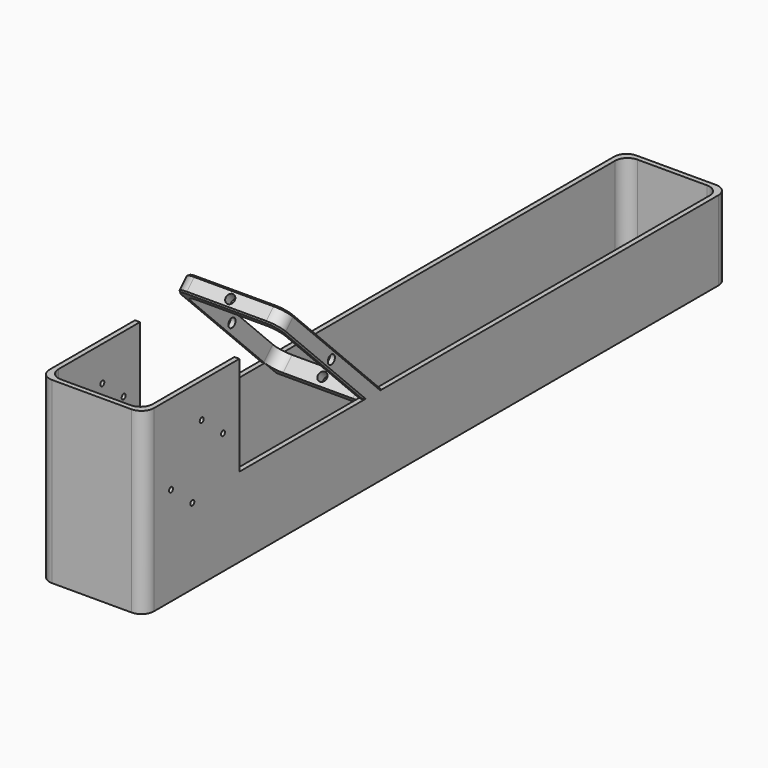
from build123d import *

# Parameters (mm, degrees)
F1_DEPTH      = 16
F3_D          = 18
F5_D          = 18
F6_ANGLE      = 45
F8_START      = -100
F8_DEPTH      = 160
F9_DEPTH      = 100
F9_DEPTH_BACK = 100
F10_T1_DEPTH  = 32
F10_T3_DEPTH  = 32
F10_T5_DEPTH  = 360
F10_T7_DEPTH  = 160
F10_T9_DEPTH  = 157
F10_T11_DEPTH = 157
F10_T13_DEPTH = 485
F10_T15_DEPTH = 285
F11_SIZE      = 3
F13_D         = 10


# Not quite as in the source:
# - a fillet or chamfer that OpenCascade refuses, or shapes differently, is made with other operations: its cross-section is extruded or revolved along the edge and cut away or added


with BuildPart() as f1:
    # F0 (on Front) → F1 (new body, symmetric)
    with BuildSketch(Plane.XZ):
        Polygon((-95, 16), (-105, 16), (-105, -16), (-105, -174), (105, -174), (105, -16), (105, 16), (95, 16), (95, -16), (95, -154), (-95, -154), (-95, -16), align=None)
        Polygon((-105, 174), (-105, 16), (-95, 16), (-95, 154), (95, 154), (95, 16), (105, 16), (105, 174), align=None)
    extrude(amount=F1_DEPTH, both=True)

    # F3 (through all)
    with Locations(Plane.YZ.offset(105)):
        with Locations((0, 0)):
            Hole(F3_D / 2)

    # F5 (through all)
    with Locations(Plane.XY.offset(174)):
        with Locations((0, 0)):
            Hole(F5_D / 2)


with BuildPart() as f1_1:
    # F6: moved
    add(f1.part.rotate(Axis((0, 0, 16), (1, 0, 0)), F6_ANGLE))

    # F7 (on Top) → F8 (join)
    with BuildSketch(Plane.XY.offset(F8_START)):
        Polygon((0, 1010), (-105, 1010), (-105, -220), (-95, -220), (-95, 1000), (0, 1000), (95, 1000), (95, -220), (105, -220), (105, 1010), align=None)
        Polygon((-95, -220), (-105, -220), (-105, -460), (0, -460), (105, -460), (105, -220), (95, -220), (95, -450), (0, -450), (-95, -450), align=None)
    extrude(amount=-F8_DEPTH)

    # F7 (on Top) → F9 (join, two sides)
    with BuildSketch(Plane.XY) as f9_sk:
        Polygon((-95, -220), (-105, -220), (-105, -460), (0, -460), (105, -460), (105, -220), (95, -220), (95, -450), (0, -450), (-95, -450), align=None)
    extrude(amount=F9_DEPTH)
    extrude(f9_sk.sketch, amount=-F9_DEPTH_BACK)

    # F10: fillet of radius 25 on 14 edges, made by hand

    # F10_s2 → F10_t1 (join)
    with BuildSketch(Plane(origin=(0, -3.313708499, -3.313708499), x_dir=(1, 0, 0), z_dir=(0, 0.7071067812, 0.7071067812))):
        with BuildLine():
            ThreePointArc((-95, 133.686291501), (-87.6776695297, 151.3639610307), (-70, 158.686291501))
            Line((-70, 158.686291501), (-95, 158.686291501))
            Line((-95, 158.686291501), (-95, 133.686291501))
        make_face()
    extrude(amount=F10_T1_DEPTH)

    # F10_s4 → F10_t3 (join)
    with BuildSketch(Plane(origin=(0, 19.313708499, 19.313708499), x_dir=(1, 0, 0), z_dir=(0, -0.7071067812, -0.7071067812))):
        with BuildLine():
            ThreePointArc((70, -158.686291501), (87.6776695297, -151.3639610307), (95, -133.686291501))
            Line((95, -133.686291501), (95, -158.686291501))
            Line((95, -158.686291501), (70, -158.686291501))
        make_face()
        with BuildLine():
            ThreePointArc((95, 124.313708499), (87.6776695297, 141.9913780286), (70, 149.313708499))
            Line((70, 149.313708499), (95, 149.313708499))
            Line((95, 149.313708499), (95, 124.313708499))
        make_face()
        with BuildLine():
            ThreePointArc((-95, 124.313708499), (-87.6776695297, 141.9913780286), (-70, 149.313708499))
            Line((-70, 149.313708499), (-95, 149.313708499))
            Line((-95, 149.313708499), (-95, 124.313708499))
        make_face()
    extrude(amount=F10_T3_DEPTH)

    # F10_s6 → F10_t5 (join)
    with BuildSketch(Plane.XY.offset(-260)):
        with BuildLine():
            ThreePointArc((-95, -425), (-87.6776695297, -442.6776695297), (-70, -450))
            Line((-70, -450), (-95, -450))
            Line((-95, -450), (-95, -425))
        make_face()
        with BuildLine():
            ThreePointArc((95, -425), (87.6776695297, -442.6776695297), (70, -450))
            Line((70, -450), (95, -450))
            Line((95, -450), (95, -425))
        make_face()
    extrude(amount=F10_T5_DEPTH)

    # F10_s8 → F10_t7 (join)
    with BuildSketch(Plane.XY.offset(-260)):
        with BuildLine():
            ThreePointArc((95, 975), (87.6776695297, 992.6776695297), (70, 1000))
            Line((70, 1000), (95, 1000))
            Line((95, 1000), (95, 975))
        make_face()
        with BuildLine():
            ThreePointArc((-95, 975), (-87.6776695297, 992.6776695297), (-70, 1000))
            Line((-70, 1000), (-95, 1000))
            Line((-95, 1000), (-95, 975))
        make_face()
    extrude(amount=F10_T7_DEPTH)

    # F10_s10 → F10_t9 (cut)
    with BuildSketch(Plane(origin=(0, 63.5078823231, 63.5078823231), x_dir=(1, 0, 0), z_dir=(0, -0.7071067812, -0.7071067812))):
        with BuildLine():
            ThreePointArc((105, 144.313708499), (97.6776695297, 161.9913780286), (80, 169.313708499))
            Line((80, 169.313708499), (105, 169.313708499))
            Line((105, 169.313708499), (105, 144.313708499))
        make_face()
    extrude(amount=F10_T9_DEPTH, mode=Mode.SUBTRACT)

    # F10_s12 → F10_t11 (cut)
    with BuildSketch(Plane(origin=(0, -47.5078823231, -47.5078823231), x_dir=(1, 0, 0), z_dir=(0, 0.7071067812, 0.7071067812))):
        with BuildLine():
            ThreePointArc((-105, -144.313708499), (-97.6776695297, -161.9913780286), (-80, -169.313708499))
            Line((-80, -169.313708499), (-105, -169.313708499))
            Line((-105, -169.313708499), (-105, -144.313708499))
        make_face()
    extrude(amount=F10_T11_DEPTH, mode=Mode.SUBTRACT)

    # F10_s14 → F10_t13 (cut)
    with BuildSketch(Plane.XY.offset(-322.5)):
        with BuildLine():
            ThreePointArc((-105, -435), (-97.6776695297, -452.6776695297), (-80, -460))
            Line((-80, -460), (-105, -460))
            Line((-105, -460), (-105, -435))
        make_face()
        with BuildLine():
            ThreePointArc((105, -435), (97.6776695297, -452.6776695297), (80, -460))
            Line((80, -460), (105, -460))
            Line((105, -460), (105, -435))
        make_face()
    extrude(amount=F10_T13_DEPTH, mode=Mode.SUBTRACT)

    # F10_s16 → F10_t15 (cut)
    with BuildSketch(Plane.XY.offset(-322.5)):
        with BuildLine():
            ThreePointArc((105, 985), (97.6776695297, 1002.6776695297), (80, 1010))
            Line((80, 1010), (105, 1010))
            Line((105, 1010), (105, 985))
        make_face()
        with BuildLine():
            ThreePointArc((-105, 985), (-97.6776695297, 1002.6776695297), (-80, 1010))
            Line((-80, 1010), (-105, 1010))
            Line((-105, 1010), (-105, 985))
        make_face()
    extrude(amount=F10_T15_DEPTH, mode=Mode.SUBTRACT)

    # F11
    f11_edges = [f1_1.edges().sort_by_distance(p)[0] for p in [
        (97.67767, -95.231493, 133.85891),
        (97.67767, -117.85891, 111.231493),
    ]]
    chamfer(f11_edges, length=F11_SIZE)

    # F13 (through all)
    with Locations(Plane.YZ.offset(105)):
        with Locations((-314.7462682585, 29.8209178701), (-261.1231572401, -15.1742148079), (-338.2576704025, -107.0995479822), (-391.8807814209, -62.1044153042)):
            Hole(F13_D / 2)


solid = f1_1.part
